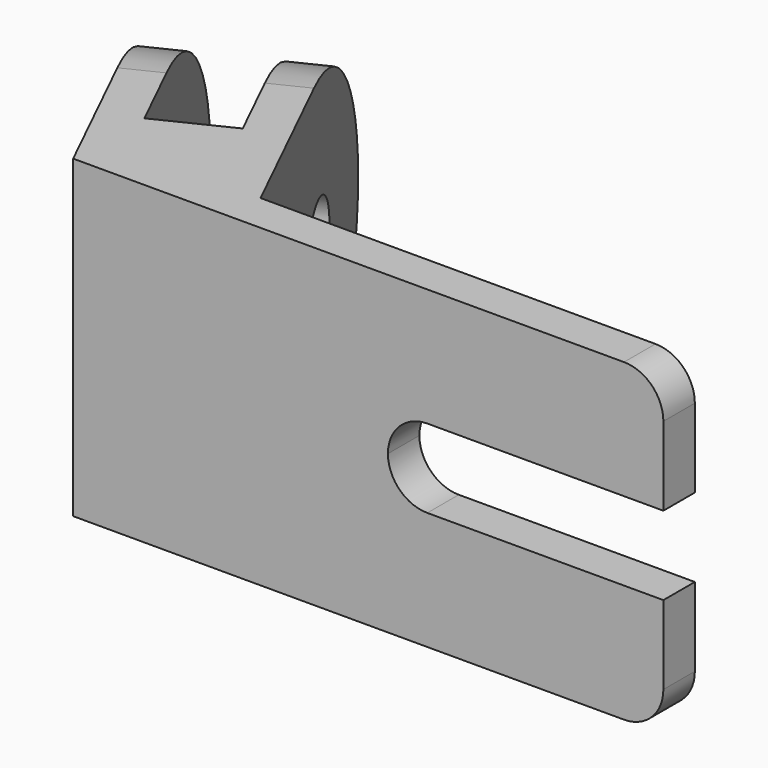
from build123d import *

# Parameters (mm, degrees)
F1_DEPTH = 80
F3_DEPTH = 25
F4_R     = 39.99999
F6_R     = 10
F7_DEPTH = 101.1
F8_R     = 10


# Not quite as in the source:
# - a fillet or chamfer is up to 0.001 mm smaller than in the source, because OpenCascade refuses the exact size


with BuildPart() as f1:
    # F0 (on Top) → F1 (new body)
    with BuildSketch(Plane.XY):
        Polygon((-75.6232507176, 0), (74.3767492824, 0), (74.3767492824, 10), (-35.9964989842, 10), (-74.7411806087, 89.4383695755), (-83.7291210717, 85.0546581076), (-57.4268522644, 31.1270153297), (-75.4027331904, 22.3595923939), (-101.7050019977, 76.2872351718), (-110.6929424607, 71.9035237039), align=None)
    extrude(amount=F1_DEPTH)

    # F2 (on face) → F3 (cut)
    with BuildSketch(Plane(origin=(0, 10, 0), x_dir=(-1, 0, 0), z_dir=(0, 1, 0))):
        with BuildLine():
            ThreePointArc((-14.3767492824, 50), (-24.3767492824, 40), (-14.3767492824, 30))
            Line((-14.3767492824, 30), (-14.3767492824, 50))
        make_face()
        with BuildLine():
            Line((-134.3767492824, 30), (-14.3767492824, 30))
            ThreePointArc((-14.3767492824, 30), (-24.3767492824, 40), (-14.3767492824, 50))
            Line((-14.3767492824, 50), (-134.3767492824, 50))
            Line((-134.3767492824, 50), (-134.3767492824, 30))
        make_face()
        with BuildLine():
            Line((-14.3767492824, 50), (-14.3767492824, 30))
            ThreePointArc((-14.3767492824, 30), (-7.3056814706, 32.9289321881), (-4.3767492824, 40))
            ThreePointArc((-4.3767492824, 40), (-7.3056814706, 47.0710678119), (-14.3767492824, 50))
        make_face()
    extrude(amount=-F3_DEPTH, mode=Mode.SUBTRACT)

    # F4 (radius 40 in the source; OpenCascade refuses exactly that, so slightly less here)
    f4_edges = [f1.edges().sort_by_distance(p)[0] for p in [
        (-79.235151, 87.246514, 80),
        (-106.198972, 74.095379, 80),
        (-106.198972, 74.095379, 0),
        (-79.235151, 87.246514, 0),
    ]]
    fillet(f4_edges, radius=F4_R)

    # F6 (on face) → F7 (cut)
    with BuildSketch(Plane(origin=(-25.1390245597, -12.2611215225, 0), x_dir=(-0.4383711468, 0.8987940463, 0), z_dir=(0.8987940463, 0.4383711468, 0))):
        with Locations((77.0729333162, 42.9970733821)):
            Circle(F6_R)
    extrude(amount=-F7_DEPTH, mode=Mode.SUBTRACT)

    # F8
    f8_edges = [f1.edges().sort_by_distance(p)[0] for p in [
        (74.376749, 5, 80),
        (74.376749, 5, 0),
    ]]
    fillet(f8_edges, radius=F8_R)


solid = f1.part
